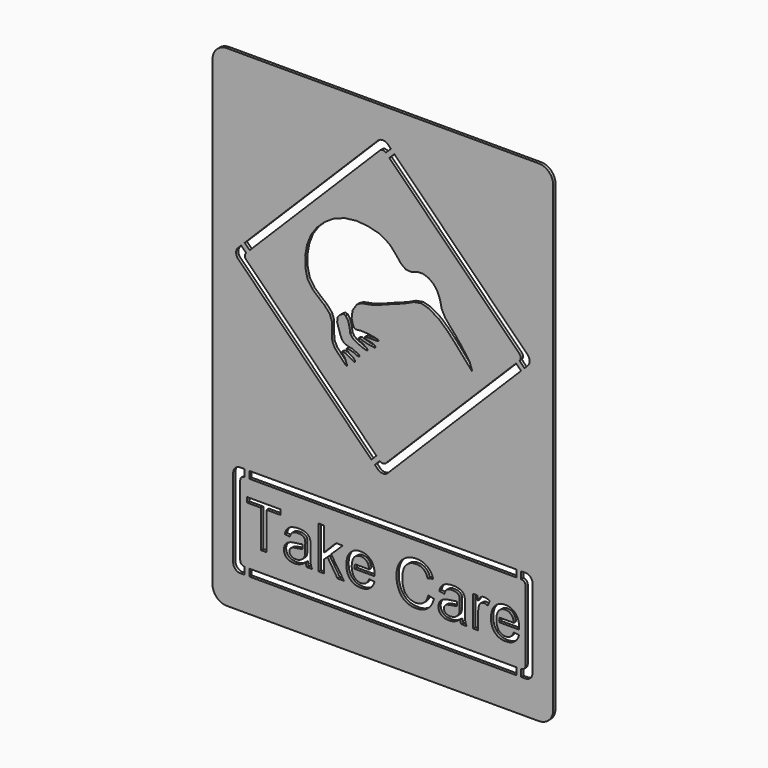
from build123d import *

# Parameters (mm, degrees)
F0_W     = 277.297216
F0_H     = 7.329178
F0_H_2   = 7.329177
F1_DEPTH = 3


# Not quite as in the source:
# - ends of sketch curves that miss each other by under 0.0002 mm in the source are joined


with BuildPart() as f1:
    # F0 (on Front) → F1 (new body)
    with BuildSketch(Plane.XZ):
        with BuildLine():
            Line((162.000001, 255), (-162, 255))
            ThreePointArc((-162, 255), (-172.6066017178, 250.6066027178), (-177, 240.000001))
            Line((-177, 240.000001), (-177, -240))
            ThreePointArc((-177, -240), (-172.6066017178, -250.6066017178), (-162, -255))
            Line((-162, -255), (162.000001, -255))
            ThreePointArc((162.000001, -255), (172.6066027178, -250.6066017178), (177.000001, -240))
            Line((177.000001, -240), (177, 240.000001))
            ThreePointArc((177, 240.000001), (172.6066027178, 250.6066027178), (162.000001, 255))
        make_face()
        with BuildLine():
            ThreePointArc((-148.146114, -208.902383), (-146.8581143129, -212.0118893129), (-143.748608, -213.299889))
            Line((-143.748608, -213.299889), (-143.748608, -220.629066))
            Line((-143.748608, -220.629066), (-148.146114, -220.629065))
            ThreePointArc((-148.146114, -220.629065), (-153.3286240501, -218.4823980501), (-155.47529, -213.299888))
            Line((-155.47529, -213.299888), (-155.47529, -131.21311))
            ThreePointArc((-155.47529, -131.21311), (-153.3286240501, -126.0305999499), (-148.146114, -123.883934))
            Line((-148.146114, -123.883934), (-143.748608, -123.883933))
            Line((-143.748608, -123.883933), (-143.748608, -131.21311))
            ThreePointArc((-143.748608, -131.21311), (-146.8581143129, -132.5011096871), (-148.146114, -135.610616))
            Line((-148.146114, -135.610616), (-148.146114, -208.902383))
        make_face(mode=Mode.SUBTRACT)
        Polygon((-120.79643, -153.786395), (-120.79643, -192.572038), (-126.615776, -192.572038), (-126.615776, -153.786395), (-141.104149, -153.786395), (-141.104149, -148.596979), (-106.248064, -148.596979), (-106.248064, -153.786395), align=None, mode=Mode.SUBTRACT)
        with Locations((0, -216.964477)):
            Rectangle(F0_W, F0_H, mode=Mode.SUBTRACT)
        Polygon((-80.02351, -189.731733), (-80.111626, -189.196011), (-80.180993, -188.64248), (-80.927393, -189.256473), (-81.666763, -189.823597), (-82.399102, -190.343851), (-83.124412, -190.817235), (-83.842691, -191.24375), (-84.553939, -191.623395), (-85.258156, -191.95617), (-85.955344, -192.242075), (-86.655343, -192.488142), (-87.367998, -192.701398), (-88.093306, -192.881848), (-88.831271, -193.029487), (-89.581889, -193.144318), (-90.345163, -193.22634), (-91.121092, -193.275553), (-91.909675, -193.291958), (-92.55636, -193.28194), (-93.184063, -193.251884), (-93.792784, -193.201792), (-94.382522, -193.131663), (-94.953279, -193.041497), (-95.505053, -192.931295), (-96.037844, -192.801056), (-96.551653, -192.65078), (-97.046481, -192.480466), (-97.522326, -192.290117), (-97.979188, -192.079731), (-98.417069, -191.849307), (-98.835967, -191.598847), (-99.235883, -191.32835), (-99.616817, -191.037816), (-99.978769, -190.727246), (-100.320215, -190.401091), (-100.639632, -190.063805), (-100.93702, -189.715386), (-101.21238, -189.355837), (-101.465711, -188.985156), (-101.697013, -188.603343), (-101.906286, -188.2104), (-102.093531, -187.806324), (-102.258747, -187.391116), (-102.401934, -186.964778), (-102.523092, -186.527307), (-102.622222, -186.078706), (-102.699323, -185.618972), (-102.754395, -185.148107), (-102.787438, -184.66611), (-102.798452, -184.172982), (-102.781813, -183.594375), (-102.731897, -183.028423), (-102.648703, -182.475126), (-102.532232, -181.934483), (-102.382483, -181.406496), (-102.199457, -180.891163), (-101.983152, -180.388485), (-101.733572, -179.898462), (-101.45704, -179.426719), (-101.159886, -178.978878), (-100.842109, -178.554941), (-100.50371, -178.154908), (-100.144687, -177.778778), (-99.765043, -177.426553), (-99.364775, -177.09823), (-98.943885, -176.793811), (-98.505888, -176.510249), (-98.054297, -176.244497), (-97.589115, -175.996557), (-97.110341, -175.766426), (-96.617975, -175.554106), (-96.112016, -175.359597), (-95.592465, -175.182898), (-95.059321, -175.02401), (-94.636556, -174.919491), (-94.163172, -174.815909), (-93.639168, -174.713263), (-93.064546, -174.611556), (-92.439303, -174.510786), (-91.763442, -174.410953), (-91.03696, -174.312058), (-90.259861, -174.2141), (-89.455927, -174.11544), (-88.678944, -174.014435), (-87.928911, -173.911088), (-87.205829, -173.805397), (-86.509696, -173.697362), (-85.840513, -173.586984), (-85.19828, -173.474262), (-84.582998, -173.359197), (-83.994666, -173.241788), (-83.685093, -173.175751), (-83.689838, -177.545451), (-83.765824, -177.564818), (-84.305529, -177.69371), (-84.8682, -177.819789), (-85.453838, -177.943057), (-86.062442, -178.063512), (-86.694011, -178.181155), (-87.348547, -178.295986), (-88.026049, -178.408005), (-88.726517, -178.517211), (-89.449951, -178.623605), (-90.251893, -178.745467), (-90.992903, -178.871078), (-91.672983, -179.000438), (-92.292132, -179.133548), (-92.850351, -179.270408), (-93.347639, -179.411017), (-93.783996, -179.555375), (-94.159422, -179.703484), (-94.494541, -179.862138), (-94.809974, -180.038134), (-95.105723, -180.231472), (-95.381785, -180.442151), (-95.638163, -180.670172), (-95.874855, -180.915535), (-96.091862, -181.17824), (-96.289183, -181.458287), (-96.464944, -181.750989), (-96.617271, -182.051658), (-96.746163, -182.360295), (-96.85162, -182.6769), (-96.933642, -183.001473), (-96.992229, -183.334013), (-97.027381, -183.674522), (-97.039099, -184.022999), (-97.013555, -184.551689), (-96.936923, -185.057883), (-96.809202, -185.541578), (-96.630394, -186.002776), (-96.400499, -186.441477), (-96.119515, -186.857681), (-95.787443, -187.251386), (-95.404283, -187.622594), (-94.971909, -187.960057), (-94.492198, -188.252524), (-93.965148, -188.499996), (-93.390759, -188.702473), (-92.769031, -188.859955), (-92.099966, -188.972443), (-91.383562, -189.039935), (-90.61982, -189.062433), (-89.850688, -189.041107), (-89.103116, -188.97713), (-88.377103, -188.870501), (-87.672651, -188.721221), (-86.989759, -188.529289), (-86.328427, -188.294707), (-85.688655, -188.017472), (-85.070444, -187.697586), (-84.483165, -187.340673), (-83.936195, -186.952357), (-83.429534, -186.532638), (-82.96318, -186.081518), (-82.537134, -185.598994), (-82.151396, -185.085067), (-81.805966, -184.539738), (-81.500844, -183.963005), (-81.296961, -183.478373), (-81.120262, -182.93937), (-80.970747, -182.345999), (-80.848418, -181.69826), (-80.753272, -180.996152), (-80.685311, -180.239674), (-80.644534, -179.428827), (-80.630943, -178.563612), (-80.623912, -172.089495), (-80.617818, -171.849991), (-80.612663, -171.635796), (-80.608444, -171.446912), (-80.605164, -171.283336), (-80.60282, -171.14507), (-80.601415, -171.032115), (-80.600945, -170.944468), (-80.606922, -170.539631), (-80.624849, -170.150026), (-80.654729, -169.775654), (-80.69656, -169.416515), (-80.750343, -169.072608), (-80.816078, -168.743934), (-80.893764, -168.430492), (-80.983402, -168.132284), (-81.084992, -167.849308), (-81.198535, -167.581565), (-81.324028, -167.329053), (-81.461473, -167.091776), (-81.610871, -166.86973), (-81.772221, -166.662918), (-81.945521, -166.471337), (-82.130774, -166.294991), (-82.397345, -166.073414), (-82.679619, -165.866132), (-82.977592, -165.673146), (-83.291268, -165.494455), (-83.620645, -165.330059), (-83.965723, -165.179959), (-84.326503, -165.044155), (-84.702984, -164.922644), (-85.095167, -164.81543), (-85.503051, -164.722511), (-85.926637, -164.643887), (-86.365923, -164.579558), (-86.82091, -164.529525), (-87.2916, -164.493786), (-87.777991, -164.472344), (-88.280083, -164.465195), (-88.748487, -164.47041), (-89.201308, -164.486053), (-89.638543, -164.512125), (-90.060195, -164.548624), (-90.466263, -164.595552), (-90.856746, -164.652909), (-91.231645, -164.720694), (-91.590961, -164.798909), (-91.934692, -164.887551), (-92.262839, -164.986621), (-92.575401, -165.096121), (-92.87238, -165.216049), (-93.153773, -165.346405), (-93.419583, -165.48719), (-93.66981, -165.638403), (-93.904451, -165.800046), (-94.127609, -165.974929), (-94.343386, -166.165864), (-94.55178, -166.372852), (-94.752794, -166.595894), (-94.946424, -166.834988), (-95.132672, -167.090136), (-95.311539, -167.361335), (-95.483024, -167.648588), (-95.647127, -167.951894), (-95.803847, -168.271253), (-95.953186, -168.606665), (-96.095142, -168.958129), (-96.229717, -169.325646), (-96.35691, -169.709216), (-96.476721, -170.108839), (-96.58915, -170.524516), (-101.868556, -169.804597), (-101.674046, -168.97758), (-101.450479, -168.19134), (-101.19785, -167.445877), (-100.916163, -166.74119), (-100.605417, -166.07728), (-100.265611, -165.454148), (-99.896746, -164.871791), (-99.498823, -164.330211), (-99.063402, -163.824018), (-98.58205, -163.347821), (-98.054766, -162.901621), (-97.48155, -162.485418), (-96.8624, -162.099212), (-96.197319, -161.743002), (-95.486304, -161.416789), (-94.729358, -161.120572), (-93.933979, -160.856929), (-93.107665, -160.628439), (-92.250418, -160.435102), (-91.362236, -160.276916), (-90.443121, -160.153883), (-89.493072, -160.066003), (-88.512088, -160.013274), (-87.50017, -159.995698), (-86.504188, -160.010696), (-85.556014, -160.055692), (-84.655646, -160.130683), (-83.803085, -160.235671), (-82.998332, -160.370656), (-82.241386, -160.535637), (-81.532247, -160.730615), (-80.870915, -160.95559), (-80.254578, -161.203297), (-79.680424, -161.46647), (-79.148452, -161.74511), (-78.658663, -162.039218), (-78.211058, -162.348793), (-77.805634, -162.673835), (-77.442394, -163.014343), (-77.121337, -163.370319), (-76.832619, -163.74598), (-76.566399, -164.145545), (-76.322676, -164.569012), (-76.101451, -165.016384), (-75.902723, -165.487659), (-75.726493, -165.982838), (-75.57276, -166.50192), (-75.441525, -167.044906), (-75.378251, -167.424551), (-75.323413, -167.873563), (-75.277012, -168.391942), (-75.239048, -168.979689), (-75.20952, -169.636802), (-75.188429, -170.363283), (-75.175773, -171.159131), (-75.171556, -172.024347), (-75.171556, -179.223538), (-75.170208, -180.143064), (-75.166165, -181.019352), (-75.159428, -181.852403), (-75.149995, -182.642217), (-75.137868, -183.388792), (-75.123046, -184.092131), (-75.105528, -184.752233), (-75.085315, -185.369098), (-75.062408, -185.942724), (-75.036805, -186.473114), (-75.008508, -186.960266), (-74.977515, -187.404181), (-74.943827, -187.804859), (-74.907444, -188.1623), (-74.868367, -188.476502), (-74.826594, -188.747468), (-74.729808, -189.243584), (-74.611931, -189.734545), (-74.472962, -190.220349), (-74.312901, -190.700999), (-74.13175, -191.176492), (-73.929508, -191.64683), (-73.706173, -192.112012), (-73.461747, -192.572038), (-79.101114, -192.572038), (-79.301716, -192.14318), (-79.483571, -191.696512), (-79.646677, -191.232032), (-79.791037, -190.749743), (-79.916648, -190.249643), align=None, mode=Mode.SUBTRACT)
        Polygon((-61.373106, -179.943457), (-61.373106, -192.572038), (-66.772499, -192.572038), (-66.772499, -148.596979), (-61.373106, -148.596979), (-61.373106, -173.674161), (-48.594541, -160.715617), (-41.605326, -160.715617), (-53.783958, -172.534289), (-40.375464, -192.572038), (-47.034716, -192.572038), (-57.563533, -176.283868), align=None, mode=Mode.SUBTRACT)
        with BuildLine():
            ThreePointArc((-29.2375033056, -178.0236729382), (-29.2848390712, -175.7969741165), (-29.0319847673, -173.5841720427))
            Line((-29.0319847673, -173.5841720427), (-14.218403, -173.584172))
            Line((-14.218403, -173.584172), (-14.268553, -173.089579))
            Line((-14.268553, -173.089579), (-14.329015, -172.610687))
            Line((-14.329015, -172.610687), (-14.399788, -172.147497))
            Line((-14.399788, -172.147497), (-14.480873, -171.700008))
            Line((-14.480873, -171.700008), (-14.572269, -171.268221))
            Line((-14.572269, -171.268221), (-14.673977, -170.852134))
            Line((-14.673977, -170.852134), (-14.785995, -170.45175))
            Line((-14.785995, -170.45175), (-14.908325, -170.067067))
            Line((-14.908325, -170.067067), (-15.040966, -169.698084))
            Line((-15.040966, -169.698084), (-15.183919, -169.344804))
            Line((-15.183919, -169.344804), (-15.337183, -169.007225))
            Line((-15.337183, -169.007225), (-15.500758, -168.685346))
            Line((-15.500758, -168.685346), (-15.674646, -168.37917))
            Line((-15.674646, -168.37917), (-15.858843, -168.088695))
            Line((-15.858843, -168.088695), (-16.053352, -167.813922))
            Line((-16.053352, -167.813922), (-16.258173, -167.554849))
            Line((-16.258173, -167.554849), (-16.586613, -167.177079))
            Line((-16.586613, -167.177079), (-16.927005, -166.823681))
            Line((-16.927005, -166.823681), (-17.279347, -166.494656))
            Line((-17.279347, -166.494656), (-17.643642, -166.190002))
            Line((-17.643642, -166.190002), (-18.01989, -165.909721))
            Line((-18.01989, -165.909721), (-18.408088, -165.653813))
            Line((-18.408088, -165.653813), (-18.808239, -165.422276))
            Line((-18.808239, -165.422276), (-19.220341, -165.215112))
            Line((-19.220341, -165.215112), (-19.644395, -165.032319))
            Line((-19.644395, -165.032319), (-20.0804, -164.8739))
            Line((-20.0804, -164.8739), (-20.528357, -164.739853))
            Line((-20.528357, -164.739853), (-20.988267, -164.630177))
            Line((-20.988267, -164.630177), (-21.460128, -164.544875))
            Line((-21.460128, -164.544875), (-21.943941, -164.483944))
            Line((-21.943941, -164.483944), (-22.439706, -164.447385))
            Line((-22.439706, -164.447385), (-22.947422, -164.435199))
            Line((-22.947422, -164.435199), (-23.407741, -164.444925))
            Line((-23.407741, -164.444925), (-23.858804, -164.474101))
            Line((-23.858804, -164.474101), (-24.30061, -164.522728))
            Line((-24.30061, -164.522728), (-24.733158, -164.590806))
            Line((-24.733158, -164.590806), (-25.156451, -164.678336))
            Line((-25.156451, -164.678336), (-25.570487, -164.785316))
            Line((-25.570487, -164.785316), (-25.975265, -164.911747))
            Line((-25.975265, -164.911747), (-26.370788, -165.05763))
            Line((-26.370788, -165.05763), (-26.757053, -165.222963))
            Line((-26.757053, -165.222963), (-27.134061, -165.407746))
            Line((-27.134061, -165.407746), (-27.501813, -165.611981))
            Line((-27.501813, -165.611981), (-27.860307, -165.835667))
            Line((-27.860307, -165.835667), (-28.209546, -166.078804))
            Line((-28.209546, -166.078804), (-28.549527, -166.341392))
            Line((-28.549527, -166.341392), (-28.880252, -166.62343))
            Line((-28.880252, -166.62343), (-29.201719, -166.924919))
            Line((-29.201719, -166.924919), (-29.509712, -167.242696))
            Line((-29.509712, -167.242696), (-29.800011, -167.573596))
            Line((-29.800011, -167.573596), (-30.072618, -167.917621))
            Line((-30.072618, -167.917621), (-30.32753, -168.274768))
            Line((-30.32753, -168.274768), (-30.564749, -168.645039))
            Line((-30.564749, -168.645039), (-30.784276, -169.028434))
            Line((-30.784276, -169.028434), (-30.986108, -169.424952))
            Line((-30.986108, -169.424952), (-31.170248, -169.834593))
            ThreePointArc((-31.170248, -169.834593), (-32.3623662835, -176.4885053369), (-31.2191093274, -183.1509867594))
            Line((-31.2191093274, -183.1509867594), (-30.773847, -184.079008))
            Line((-30.773847, -184.079008), (-30.523445, -184.514194))
            Line((-30.523445, -184.514194), (-30.254531, -184.930162))
            Line((-30.254531, -184.930162), (-29.967102, -185.326915))
            Line((-29.967102, -185.326915), (-29.66116, -185.70445))
            Line((-29.66116, -185.70445), (-29.336704, -186.062769))
            Line((-29.336704, -186.062769), (-28.997836, -186.400583))
            Line((-28.997836, -186.400583), (-28.648657, -186.716603))
            Line((-28.648657, -186.716603), (-28.289166, -187.010828))
            Line((-28.289166, -187.010828), (-27.919363, -187.283257))
            Line((-27.919363, -187.283257), (-27.53925, -187.533894))
            Line((-27.53925, -187.533894), (-27.148824, -187.762735))
            Line((-27.148824, -187.762735), (-26.748089, -187.969782))
            Line((-26.748089, -187.969782), (-26.337041, -188.155035))
            Line((-26.337041, -188.155035), (-25.915682, -188.318493))
            Line((-25.915682, -188.318493), (-25.484012, -188.460157))
            Line((-25.484012, -188.460157), (-25.042031, -188.580026))
            Line((-25.042031, -188.580026), (-24.589737, -188.678101))
            Line((-24.589737, -188.678101), (-24.127134, -188.754381))
            Line((-24.127134, -188.754381), (-23.654218, -188.808867))
            Line((-23.654218, -188.808867), (-23.170991, -188.841559))
            Line((-23.170991, -188.841559), (-22.677452, -188.852456))
            Line((-22.677452, -188.852456), (-21.948628, -188.828084))
            Line((-21.948628, -188.828084), (-21.246988, -188.754967))
            Line((-21.246988, -188.754967), (-20.572533, -188.633106))
            Line((-20.572533, -188.633106), (-19.925261, -188.4625))
            Line((-19.925261, -188.4625), (-19.305174, -188.24315))
            Line((-19.305174, -188.24315), (-18.712273, -187.975055))
            Line((-18.712273, -187.975055), (-18.146555, -187.658216))
            Line((-18.146555, -187.658216), (-17.608022, -187.292631))
            Line((-17.608022, -187.292631), (-17.096672, -186.873616))
            Line((-17.096672, -186.873616), (-16.612509, -186.396483))
            Line((-16.612509, -186.396483), (-16.155529, -185.861229))
            Line((-16.155529, -185.861229), (-15.725733, -185.267859))
            Line((-15.725733, -185.267859), (-15.323122, -184.616369))
            Line((-15.323122, -184.616369), (-14.947696, -183.906762))
            Line((-14.947696, -183.906762), (-14.599453, -183.139035))
            Line((-14.599453, -183.139035), (-14.278396, -182.313191))
            Line((-14.278396, -182.313191), (-8.699023, -183.003113))
            Line((-8.699023, -183.003113), (-8.872792, -183.605741))
            Line((-8.872792, -183.605741), (-9.064138, -184.191261))
            Line((-9.064138, -184.191261), (-9.273059, -184.759674))
            Line((-9.273059, -184.759674), (-9.499557, -185.310979))
            Line((-9.499557, -185.310979), (-9.743632, -185.845177))
            Line((-9.743632, -185.845177), (-10.005281, -186.362268))
            Line((-10.005281, -186.362268), (-10.284509, -186.86225))
            Line((-10.284509, -186.86225), (-10.581311, -187.345125))
            Line((-10.581311, -187.345125), (-10.895689, -187.810893))
            Line((-10.895689, -187.810893), (-11.227644, -188.259554))
            Line((-11.227644, -188.259554), (-11.577176, -188.691107))
            Line((-11.577176, -188.691107), (-11.944283, -189.105553))
            Line((-11.944283, -189.105553), (-12.328966, -189.502891))
            Line((-12.328966, -189.502891), (-12.731225, -189.883122))
            Line((-12.731225, -189.883122), (-13.151061, -190.246245))
            Line((-13.151061, -190.246245), (-13.588473, -190.592261))
            Line((-13.588473, -190.592261), (-14.042407, -190.919177))
            Line((-14.042407, -190.919177), (-14.511807, -191.225003))
            Line((-14.511807, -191.225003), (-14.996674, -191.509736))
            Line((-14.996674, -191.509736), (-15.497008, -191.773378))
            Line((-15.497008, -191.773378), (-16.01281, -192.015929))
            Line((-16.01281, -192.015929), (-16.544078, -192.237388))
            Line((-16.544078, -192.237388), (-17.090815, -192.437757))
            Line((-17.090815, -192.437757), (-17.653017, -192.617033))
            Line((-17.653017, -192.617033), (-18.230686, -192.775219))
            Line((-18.230686, -192.775219), (-18.823823, -192.912313))
            Line((-18.823823, -192.912313), (-19.432426, -193.028316))
            Line((-19.432426, -193.028316), (-20.056496, -193.123227))
            Line((-20.056496, -193.123227), (-20.696034, -193.197046))
            Line((-20.696034, -193.197046), (-21.351038, -193.249775))
            Line((-21.351038, -193.249775), (-22.02151, -193.281412))
            Line((-22.02151, -193.281412), (-22.707449, -193.291958))
            Line((-22.707449, -193.291958), (-23.569793, -193.275143))
            Line((-23.569793, -193.275143), (-24.409524, -193.224699))
            Line((-24.409524, -193.224699), (-25.226638, -193.140627))
            Line((-25.226638, -193.140627), (-26.021139, -193.022925))
            Line((-26.021139, -193.022925), (-26.793025, -192.871595))
            Line((-26.793025, -192.871595), (-27.542297, -192.686635))
            Line((-27.542297, -192.686635), (-28.268953, -192.468046))
            Line((-28.268953, -192.468046), (-28.972995, -192.215828))
            Line((-28.972995, -192.215828), (-29.654423, -191.929982))
            Line((-29.654423, -191.929982), (-30.313235, -191.610505))
            Line((-30.313235, -191.610505), (-30.949433, -191.257401))
            Line((-30.949433, -191.257401), (-31.563016, -190.870667))
            Line((-31.563016, -190.870667), (-32.153985, -190.450304))
            Line((-32.153985, -190.450304), (-32.722339, -189.996313))
            Line((-32.722339, -189.996313), (-33.268079, -189.508691))
            Line((-33.268079, -189.508691), (-33.791204, -188.987441))
            Line((-33.791204, -188.987441), (-34.287027, -188.435843))
            Line((-34.287027, -188.435843), (-34.750862, -187.857178))
            Line((-34.750862, -187.857178), (-35.182708, -187.251445))
            Line((-35.182708, -187.251445), (-35.582565, -186.618645))
            Line((-35.582565, -186.618645), (-35.950434, -185.958777))
            Line((-35.950434, -185.958777), (-36.286314, -185.271843))
            Line((-36.286314, -185.271843), (-36.590206, -184.557841))
            Line((-36.590206, -184.557841), (-36.862109, -183.816772))
            Line((-36.862109, -183.816772), (-37.102023, -183.048636))
            Line((-37.102023, -183.048636), (-37.309949, -182.253432))
            Line((-37.309949, -182.253432), (-37.485886, -181.431161))
            Line((-37.485886, -181.431161), (-37.629835, -180.581823))
            Line((-37.629835, -180.581823), (-37.741795, -179.705417))
            Line((-37.741795, -179.705417), (-37.821767, -178.801945))
            Line((-37.821767, -178.801945), (-37.86975, -177.871404))
            Line((-37.86975, -177.871404), (-37.885744, -176.913798))
            Line((-37.885744, -176.913798), (-37.869574, -175.922972))
            Line((-37.869574, -175.922972), (-37.821064, -174.960267))
            Line((-37.821064, -174.960267), (-37.740214, -174.025684))
            Line((-37.740214, -174.025684), (-37.627023, -173.119223))
            Line((-37.627023, -173.119223), (-37.481493, -172.240885))
            Line((-37.481493, -172.240885), (-37.303622, -171.390668))
            Line((-37.303622, -171.390668), (-37.093411, -170.568572))
            Line((-37.093411, -170.568572), (-36.85086, -169.774599))
            Line((-36.85086, -169.774599), (-36.575969, -169.008748))
            Line((-36.575969, -169.008748), (-36.268738, -168.271018))
            Line((-36.268738, -168.271018), (-35.929167, -167.56141))
            Line((-35.929167, -167.56141), (-35.557256, -166.879925))
            Line((-35.557256, -166.879925), (-35.153004, -166.226561))
            Line((-35.153004, -166.226561), (-34.716413, -165.601318))
            Line((-34.716413, -165.601318), (-34.247481, -165.004198))
            Line((-34.247481, -165.004198), (-33.746209, -164.435199))
            Line((-33.746209, -164.435199), (-33.219159, -163.897603))
            Line((-33.219159, -163.897603), (-32.672891, -163.394691))
            Line((-32.672891, -163.394691), (-32.107409, -162.926462))
            Line((-32.107409, -162.926462), (-31.522709, -162.492917))
            Line((-31.522709, -162.492917), (-30.918792, -162.094055))
            Line((-30.918792, -162.094055), (-30.295659, -161.729878))
            Line((-30.295659, -161.729878), (-29.653309, -161.400384))
            Line((-29.653309, -161.400384), (-28.991743, -161.105573))
            Line((-28.991743, -161.105573), (-28.31096, -160.845446))
            Line((-28.31096, -160.845446), (-27.610961, -160.620002))
            Line((-27.610961, -160.620002), (-26.891745, -160.429243))
            Line((-26.891745, -160.429243), (-26.153312, -160.273167))
            Line((-26.153312, -160.273167), (-25.395663, -160.151774))
            Line((-25.395663, -160.151774), (-24.618797, -160.065065))
            Line((-24.618797, -160.065065), (-23.822715, -160.01304))
            Line((-23.822715, -160.01304), (-23.007415, -159.995698))
            Line((-23.007415, -159.995698), (-22.217895, -160.012688))
            Line((-22.217895, -160.012688), (-21.446653, -160.063659))
            Line((-21.446653, -160.063659), (-20.693691, -160.14861))
            Line((-20.693691, -160.14861), (-19.959008, -160.267542))
            Line((-19.959008, -160.267542), (-19.242603, -160.420455))
            Line((-19.242603, -160.420455), (-18.544479, -160.607348))
            Line((-18.544479, -160.607348), (-17.864633, -160.828221))
            Line((-17.864633, -160.828221), (-17.203068, -161.083075))
            Line((-17.203068, -161.083075), (-16.55978, -161.371911))
            Line((-16.55978, -161.371911), (-15.934772, -161.694725))
            Line((-15.934772, -161.694725), (-15.328043, -162.051521))
            Line((-15.328043, -162.051521), (-14.739594, -162.442298))
            Line((-14.739594, -162.442298), (-14.169423, -162.867055))
            Line((-14.169423, -162.867055), (-13.617533, -163.325792))
            Line((-13.617533, -163.325792), (-13.083921, -163.81851))
            Line((-13.083921, -163.81851), (-12.568587, -164.34521))
            Line((-12.568587, -164.34521), (-12.078213, -164.902724))
            Line((-12.078213, -164.902724), (-11.619475, -165.487893))
            Line((-11.619475, -165.487893), (-11.192375, -166.100715))
            Line((-11.192375, -166.100715), (-10.796912, -166.74119))
            Line((-10.796912, -166.74119), (-10.433086, -167.409318))
            Line((-10.433086, -167.409318), (-10.100896, -168.105099))
            Line((-10.100896, -168.105099), (-9.800344, -168.828534))
            Line((-9.800344, -168.828534), (-9.531429, -169.579621))
            Line((-9.531429, -169.579621), (-9.294151, -170.358362))
            Line((-9.294151, -170.358362), (-9.08851, -171.164755))
            Line((-9.08851, -171.164755), (-8.914506, -171.998802))
            Line((-8.914506, -171.998802), (-8.772139, -172.860502))
            Line((-8.772139, -172.860502), (-8.661409, -173.749856))
            Line((-8.661409, -173.749856), (-8.582317, -174.666862))
            Line((-8.582317, -174.666862), (-8.534862, -175.611522))
            Line((-8.534862, -175.611522), (-8.519043, -176.583835))
            Line((-8.519043, -176.583835), (-8.520917, -176.853804))
            Line((-8.520917, -176.853804), (-8.526542, -177.183767))
            Line((-8.526542, -177.183767), (-8.535915, -177.573723))
            Line((-8.535915, -177.573723), (-8.54904, -178.023673))
            Line((-8.54904, -178.023673), (-29.2375033056, -178.0236729382))
        make_face(mode=Mode.SUBTRACT)
        with Locations((0, -127.5485215)):
            Rectangle(F0_W, F0_H_2, mode=Mode.SUBTRACT)
        Polygon((46.880515, -178.498464), (47.056159, -177.836779), (47.214697, -177.15377), (53.034043, -178.623605), (52.793894, -179.506455), (52.530896, -180.362707), (52.245049, -181.19236), (51.936353, -181.995414), (51.604809, -182.77187), (51.250415, -183.521727), (50.873172, -184.244985), (50.473081, -184.941645), (50.05014, -185.611707), (49.60435, -186.25517), (49.135711, -186.872034), (48.644223, -187.4623), (48.129887, -188.025967), (47.592701, -188.563036), (47.032666, -189.073505), (46.449783, -189.557377), (45.847214, -190.013244), (45.228123, -190.439699), (44.592511, -190.836745), (43.940377, -191.204379), (43.271722, -191.542603), (42.586545, -191.851416), (41.884846, -192.130819), (41.166626, -192.38081), (40.431885, -192.601391), (39.680621, -192.792561), (38.912836, -192.95432), (38.12853, -193.086668), (37.327701, -193.189606), (36.510352, -193.263133), (35.67648, -193.307249), (34.826088, -193.321954), (33.947808, -193.310647), (33.090267, -193.276725), (32.253466, -193.220188), (31.437406, -193.141037), (30.642086, -193.039271), (29.867505, -192.914891), (29.113664, -192.767895), (28.380562, -192.598286), (27.668201, -192.406061), (26.976579, -192.191222), (26.305698, -191.953768), (25.655556, -191.6937), (25.026153, -191.411017), (24.417492, -191.105719), (23.82957, -190.777806), (23.262387, -190.427279), (22.713894, -190.055309), (22.18204, -189.663068), (21.666824, -189.250556), (21.168247, -188.817773), (20.686309, -188.364719), (20.22101, -187.891393), (19.77235, -187.397795), (19.340328, -186.883927), (18.924945, -186.349788), (18.5262, -185.795378), (18.144095, -185.220696), (17.778628, -184.625743), (17.4298, -184.01052), (17.097611, -183.375024), (16.782061, -182.719258), (16.483149, -182.043222), (16.201638, -181.353884), (15.938288, -180.658221), (15.6931, -179.956229), (15.466076, -179.247911), (15.257213, -178.533264), (15.066511, -177.81229), (14.893972, -177.084989), (14.739594, -176.35136), (14.603379, -175.611405), (14.485327, -174.865122), (14.385435, -174.11251), (14.303706, -173.353572), (14.240139, -172.588307), (14.194734, -171.816714), (14.16749, -171.038793), (14.158409, -170.254545), (14.168662, -169.402747), (14.199421, -168.564657), (14.250685, -167.740277), (14.322454, -166.929606), (14.414728, -166.132645), (14.527509, -165.349394), (14.660795, -164.579851), (14.814587, -163.824018), (14.988883, -163.081894), (15.183685, -162.35348), (15.398994, -161.638775), (15.634806, -160.937779), (15.891125, -160.250493), (16.16795, -159.576917), (16.465279, -158.917049), (16.783115, -158.270891), (17.119874, -157.641196), (17.473975, -157.030718), (17.845418, -156.439457), (18.234202, -155.867411), (18.640328, -155.314584), (19.063796, -154.780972), (19.504606, -154.266575), (19.962758, -153.771397), (20.438252, -153.295435), (20.931087, -152.83869), (21.441263, -152.401161), (21.968782, -151.982848), (22.513644, -151.583752), (23.075845, -151.203873), (23.65539, -150.843211), (24.252276, -150.501765), (24.861641, -150.180296), (25.478622, -149.879569), (26.10322, -149.599581), (26.735435, -149.340332), (27.375265, -149.101824), (28.022712, -148.884056), (28.677775, -148.687026), (29.340455, -148.510738), (30.010751, -148.355189), (30.688662, -148.22038), (31.374191, -148.106311), (32.067336, -148.012982), (32.768096, -147.940392), (33.476474, -147.888542), (34.192468, -147.857433), (34.916078, -147.847063), (35.732783, -147.860186), (36.533084, -147.899557), (37.31698, -147.965175), (38.084472, -148.057039), (38.835559, -148.175151), (39.570243, -148.319509), (40.288522, -148.490115), (40.990396, -148.686968), (41.675865, -148.910068), (42.344931, -149.159415), (42.997592, -149.435009), (43.633848, -149.73685), (44.253701, -150.064938), (44.857149, -150.419274), (45.444192, -150.799856), (46.014831, -151.206686), (46.566605, -151.637301), (47.097053, -152.089243), (47.606176, -152.562509), (48.093973, -153.057102), (48.560444, -153.573021), (49.00559, -154.110266), (49.429409, -154.668835), (49.831903, -155.248731), (50.213071, -155.849953), (50.572913, -156.4725), (50.91143, -157.116373), (51.22862, -157.781572), (51.524486, -158.468096), (51.799025, -159.175947), (52.052239, -159.905122), (52.284127, -160.655624), (46.55477, -162.005473), (46.358152, -161.415734), (46.150753, -160.846383), (45.932575, -160.297422), (45.703616, -159.768848), (45.463877, -159.260664), (45.213359, -158.772866), (44.95206, -158.305458), (44.679982, -157.858438), (44.397122, -157.431806), (44.103484, -157.025563), (43.799065, -156.639707), (43.483865, -156.274241), (43.157887, -155.929162), (42.821128, -155.604473), (42.473588, -155.300171), (42.115269, -155.016257), (41.745702, -154.751092), (41.364417, -154.503034), (40.971414, -154.272083), (40.566693, -154.058239), (40.150256, -153.861504), (39.7221, -153.681876), (39.282228, -153.519355), (38.830639, -153.373942), (38.367331, -153.245636), (37.892306, -153.134438), (37.405564, -153.040347), (36.907104, -152.963363), (36.396927, -152.903487), (35.875033, -152.860719), (35.341421, -152.835057), (34.796092, -152.826504), (34.168916, -152.835995), (33.554747, -152.864468), (32.953583, -152.911924), (32.365427, -152.978361), (31.790277, -153.063781), (31.228133, -153.168183), (30.678996, -153.291569), (30.142864, -153.433935), (29.61974, -153.595284), (29.10962, -153.775616), (28.612509, -153.974929), (28.128403, -154.193225), (27.657304, -154.430503), (27.19921, -154.686763), (26.754124, -154.962005), (26.322043, -155.25623), (25.904376, -155.566449), (25.502526, -155.889675), (25.116495, -156.225907), (24.746283, -156.575144), (24.391889, -156.937389), (24.053314, -157.31264), (23.730558, -157.700897), (23.423619, -158.102161), (23.132499, -158.516431), (22.857198, -158.943707), (22.597716, -159.383989), (22.354051, -159.837278), (22.126206, -160.303574), (21.914179, -160.782875), (21.717971, -161.275183), (21.537581, -161.780497), (21.21418, -162.808117), (20.933899, -163.843703), (20.696738, -164.887258), (20.502697, -165.93878), (20.351777, -166.998271), (20.243976, -168.065729), (20.179296, -169.141155), (20.157736, -170.224549), (20.18328, -171.604628), (20.259912, -172.940182), (20.387632, -174.231208), (20.56644, -175.477709), (20.796336, -176.679683), (21.07732, -177.837131), (21.409393, -178.950053), (21.792553, -180.018449), (22.003993, -180.533254), (22.229612, -181.031538), (22.46941, -181.5133), (22.723385, -181.978541), (22.991539, -182.42726), (23.27387, -182.859457), (23.57038, -183.275134), (23.881068, -183.674288), (24.205934, -184.056921), (24.544978, -184.423032), (24.8982, -184.772621), (25.265599, -185.10569), (25.647177, -185.422236), (26.042934, -185.722261), (26.452868, -186.005765), (26.876981, -186.272746), (27.74829, -186.757848), (28.637408, -187.17827), (29.544337, -187.534011), (30.469077, -187.825071), (31.411628, -188.051452), (32.371988, -188.213153), (33.35016, -188.310173), (34.346142, -188.342513), (34.951464, -188.331499), (35.54507, -188.298456), (36.126957, -188.243384), (36.697128, -188.166284), (37.255581, -188.067154), (37.802316, -187.945995), (38.337334, -187.802809), (38.860635, -187.637593), (39.372218, -187.450348), (39.872084, -187.241075), (40.360232, -187.009773), (40.836662, -186.756442), (41.301377, -186.481082), (41.754373, -186.183693), (42.195651, -185.864276), (42.625212, -185.52283), (43.04036, -185.159707), (43.438402, -184.775258), (43.819335, -184.369484), (44.183162, -183.942383), (44.529881, -183.493956), (44.859493, -183.024205), (45.171996, -182.533128), (45.467393, -182.020723), (45.745682, -181.486994), (46.006863, -180.93194), (46.250938, -180.355559), (46.477904, -179.757852), (46.687764, -179.138821), align=None, mode=Mode.SUBTRACT)
        Polygon((80.458463, -189.731733), (80.370347, -189.196011), (80.30098, -188.64248), (79.554579, -189.256473), (78.815209, -189.823597), (78.082869, -190.343851), (77.357561, -190.817235), (76.639282, -191.24375), (75.928034, -191.623395), (75.223815, -191.95617), (74.526628, -192.242075), (73.826629, -192.488142), (73.113975, -192.701398), (72.388665, -192.881848), (71.650701, -193.029487), (70.900082, -193.144318), (70.136809, -193.22634), (69.360881, -193.275553), (68.572298, -193.291958), (67.925612, -193.28194), (67.29791, -193.251884), (66.689189, -193.201792), (66.09945, -193.131663), (65.528694, -193.041497), (64.97692, -192.931295), (64.444128, -192.801056), (63.930318, -192.65078), (63.435492, -192.480466), (62.959647, -192.290117), (62.502783, -192.079731), (62.064904, -191.849307), (61.646005, -191.598847), (61.246089, -191.32835), (60.865155, -191.037816), (60.503204, -190.727246), (60.161758, -190.401091), (59.842341, -190.063805), (59.544952, -189.715386), (59.269593, -189.355837), (59.016261, -188.985156), (58.784959, -188.603343), (58.575685, -188.2104), (58.388441, -187.806324), (58.223226, -187.391116), (58.080039, -186.964778), (57.95888, -186.527307), (57.859751, -186.078706), (57.78265, -185.618972), (57.727578, -185.148107), (57.694535, -184.66611), (57.68352, -184.172982), (57.700159, -183.594375), (57.750075, -183.028423), (57.833269, -182.475126), (57.949741, -181.934483), (58.099489, -181.406496), (58.282516, -180.891163), (58.498819, -180.388485), (58.748401, -179.898462), (59.024932, -179.426719), (59.322087, -178.978878), (59.639864, -178.554941), (59.978263, -178.154908), (60.337285, -177.778778), (60.71693, -177.426553), (61.117197, -177.09823), (61.538088, -176.793811), (61.976085, -176.510249), (62.427675, -176.244497), (62.892857, -175.996557), (63.371632, -175.766426), (63.863998, -175.554106), (64.369957, -175.359597), (64.889508, -175.182898), (65.422651, -175.02401), (65.845416, -174.919491), (66.3188, -174.815909), (66.842804, -174.713263), (67.417427, -174.611556), (68.04267, -174.510786), (68.718531, -174.410953), (69.445012, -174.312058), (70.222112, -174.2141), (71.026045, -174.11544), (71.803028, -174.014435), (72.553061, -173.911088), (73.276144, -173.805397), (73.972276, -173.697362), (74.64146, -173.586984), (75.283691, -173.474262), (75.898974, -173.359197), (76.487307, -173.241788), (76.79688, -173.175751), (76.792134, -177.545451), (76.716148, -177.564818), (76.176443, -177.69371), (75.613772, -177.819789), (75.028135, -177.943057), (74.419531, -178.063512), (73.787961, -178.181155), (73.133425, -178.295986), (72.455923, -178.408005), (71.755455, -178.517211), (71.032021, -178.623605), (70.23008, -178.745467), (69.489069, -178.871078), (68.80899, -179.000438), (68.18984, -179.133548), (67.631622, -179.270408), (67.134334, -179.411017), (66.697976, -179.555375), (66.32255, -179.703484), (65.987432, -179.862138), (65.671998, -180.038134), (65.37625, -180.231472), (65.100187, -180.442151), (64.84381, -180.670172), (64.607118, -180.915535), (64.390111, -181.17824), (64.192789, -181.458287), (64.017027, -181.750989), (63.864701, -182.051658), (63.735809, -182.360295), (63.630353, -182.6769), (63.54833, -183.001473), (63.489744, -183.334013), (63.454591, -183.674522), (63.442874, -184.022999), (63.468417, -184.551689), (63.54505, -185.057883), (63.672769, -185.541578), (63.851577, -186.002776), (64.081474, -186.441477), (64.362458, -186.857681), (64.69453, -187.251386), (65.07769, -187.622594), (65.510063, -187.960057), (65.989775, -188.252524), (66.516825, -188.499996), (67.091214, -188.702473), (67.71294, -188.859955), (68.382006, -188.972443), (69.09841, -189.039935), (69.862153, -189.062433), (70.631285, -189.041107), (71.378857, -188.97713), (72.10487, -188.870501), (72.809321, -188.721221), (73.492213, -188.529289), (74.153546, -188.294707), (74.793317, -188.017472), (75.411529, -187.697586), (75.998806, -187.340673), (76.545776, -186.952357), (77.052439, -186.532638), (77.518792, -186.081518), (77.944838, -185.598994), (78.330576, -185.085067), (78.676006, -184.539738), (78.981128, -183.963005), (79.185011, -183.478373), (79.361711, -182.93937), (79.511224, -182.345999), (79.633555, -181.69826), (79.728701, -180.996152), (79.796661, -180.239674), (79.837438, -179.428827), (79.85103, -178.563612), (79.858061, -172.089495), (79.864153, -171.849991), (79.86931, -171.635796), (79.873528, -171.446912), (79.876809, -171.283336), (79.879153, -171.14507), (79.880558, -171.032115), (79.881027, -170.944468), (79.875051, -170.539631), (79.857124, -170.150026), (79.827244, -169.775654), (79.785413, -169.416515), (79.73163, -169.072608), (79.665895, -168.743934), (79.588209, -168.430492), (79.49857, -168.132284), (79.39698, -167.849308), (79.283438, -167.581565), (79.157944, -167.329053), (79.020498, -167.091776), (78.871101, -166.86973), (78.709752, -166.662918), (78.536451, -166.471337), (78.351199, -166.294991), (78.084627, -166.073414), (77.802354, -165.866132), (77.504379, -165.673146), (77.190704, -165.494455), (76.861328, -165.330059), (76.516248, -165.179959), (76.155469, -165.044155), (75.778988, -164.922644), (75.386805, -164.81543), (74.978922, -164.722511), (74.555336, -164.643887), (74.11605, -164.579558), (73.661061, -164.529525), (73.190372, -164.493786), (72.703982, -164.472344), (72.20189, -164.465195), (71.733486, -164.47041), (71.280665, -164.486053), (70.843428, -164.512125), (70.421777, -164.548624), (70.01571, -164.595552), (69.625226, -164.652909), (69.250326, -164.720694), (68.891012, -164.798909), (68.547281, -164.887551), (68.219134, -164.986621), (67.906571, -165.096121), (67.609593, -165.216049), (67.328198, -165.346405), (67.062388, -165.48719), (66.812163, -165.638403), (66.577521, -165.800046), (66.354363, -165.974929), (66.138587, -166.165864), (65.930192, -166.372852), (65.729179, -166.595894), (65.535548, -166.834988), (65.3493, -167.090136), (65.170433, -167.361335), (64.998949, -167.648588), (64.834846, -167.951894), (64.678125, -168.271253), (64.528787, -168.606665), (64.386829, -168.958129), (64.252255, -169.325646), (64.125063, -169.709216), (64.005252, -170.108839), (63.892823, -170.524516), (58.613416, -169.804597), (58.807925, -168.97758), (59.031494, -168.19134), (59.284122, -167.445877), (59.565809, -166.74119), (59.876556, -166.07728), (60.216361, -165.454148), (60.585226, -164.871791), (60.98315, -164.330211), (61.418569, -163.824018), (61.899922, -163.347821), (62.427207, -162.901621), (63.000423, -162.485418), (63.619572, -162.099212), (64.284654, -161.743002), (64.995668, -161.416789), (65.752614, -161.120572), (66.547993, -160.856929), (67.374306, -160.628439), (68.231554, -160.435102), (69.119736, -160.276916), (70.038851, -160.153883), (70.988901, -160.066003), (71.969885, -160.013274), (72.981802, -159.995698), (73.977783, -160.010696), (74.925958, -160.055692), (75.826326, -160.130683), (76.678886, -160.235671), (77.48364, -160.370656), (78.240586, -160.535637), (78.949726, -160.730615), (79.611057, -160.95559), (80.227394, -161.203297), (80.801549, -161.46647), (81.33352, -161.74511), (81.823308, -162.039218), (82.270915, -162.348793), (82.676338, -162.673835), (83.039579, -163.014343), (83.360636, -163.370319), (83.649354, -163.74598), (83.915574, -164.145545), (84.159296, -164.569012), (84.380522, -165.016384), (84.579249, -165.487659), (84.75548, -165.982838), (84.909212, -166.50192), (85.040447, -167.044906), (85.103721, -167.424551), (85.158559, -167.873563), (85.20496, -168.391942), (85.242925, -168.979689), (85.272453, -169.636802), (85.293544, -170.363283), (85.306199, -171.159131), (85.310417, -172.024347), (85.310417, -179.223538), (85.311764, -180.143064), (85.315807, -181.019352), (85.322545, -181.852403), (85.331977, -182.642217), (85.344105, -183.388792), (85.358927, -184.092131), (85.376445, -184.752233), (85.396657, -185.369098), (85.419565, -185.942724), (85.445167, -186.473114), (85.473465, -186.960266), (85.504458, -187.404181), (85.538145, -187.804859), (85.574528, -188.1623), (85.613606, -188.476502), (85.655378, -188.747468), (85.752165, -189.243584), (85.870042, -189.734545), (86.009011, -190.220349), (86.16907, -190.700999), (86.350222, -191.176492), (86.552465, -191.64683), (86.775799, -192.112012), (87.020225, -192.572038), (81.380859, -192.572038), (81.180256, -192.14318), (80.998402, -191.696512), (80.835294, -191.232032), (80.690936, -190.749743), (80.565325, -190.249643), align=None, mode=Mode.SUBTRACT)
        Polygon((99.018877, -175.893912), (99.018877, -192.572038), (93.619484, -192.572038), (93.619484, -160.715617), (98.478937, -160.715617), (98.478937, -165.545074), (98.710299, -165.130394), (98.939433, -164.733759), (99.166341, -164.355169), (99.391023, -163.994623), (99.613478, -163.652123), (99.833707, -163.327667), (100.05171, -163.021257), (100.267487, -162.732891), (100.481037, -162.462569), (100.692361, -162.210293), (100.901459, -161.976062), (101.10833, -161.759875), (101.312975, -161.561733), (101.515394, -161.381636), (101.715586, -161.219584), (101.913552, -161.075576), (102.312179, -160.82248), (102.720649, -160.60313), (103.138961, -160.417525), (103.567116, -160.265668), (104.005114, -160.147556), (104.452954, -160.063191), (104.910637, -160.012571), (105.378163, -159.995698), (106.061993, -160.022882), (106.748634, -160.104435), (107.438088, -160.240358), (108.130354, -160.430649), (108.825432, -160.675309), (109.523322, -160.974338), (110.224025, -161.327736), (110.92754, -161.735502), (109.067748, -166.744939), (108.572804, -166.470752), (108.077859, -166.233123), (107.582915, -166.032051), (107.087971, -165.867538), (106.593026, -165.739584), (106.098082, -165.648188), (105.603137, -165.59335), (105.108193, -165.575072), (104.671367, -165.59171), (104.24579, -165.641627), (103.831462, -165.72482), (103.428382, -165.841292), (103.036551, -165.99104), (102.655969, -166.174067), (102.286635, -166.39037), (101.928551, -166.639952), (101.588745, -166.91906), (101.274248, -167.223949), (100.985063, -167.554614), (100.721186, -167.911058), (100.482619, -168.293282), (100.269362, -168.701283), (100.081414, -169.135061), (99.918776, -169.594619), (99.707862, -170.322975), (99.525071, -171.068204), (99.3704, -171.830306), (99.243852, -172.609281), (99.145426, -173.405129), (99.075121, -174.21785), (99.032938, -175.047444), align=None, mode=Mode.SUBTRACT)
        with BuildLine():
            ThreePointArc((120.9856216944, -178.0236729382), (120.9382859288, -175.7969741165), (121.1911402327, -173.5841720427))
            Line((121.1911402327, -173.5841720427), (136.004722, -173.584172))
            Line((136.004722, -173.584172), (135.954572, -173.089579))
            Line((135.954572, -173.089579), (135.89411, -172.610687))
            Line((135.89411, -172.610687), (135.823336, -172.147497))
            Line((135.823336, -172.147497), (135.742252, -171.700008))
            Line((135.742252, -171.700008), (135.650855, -171.268221))
            Line((135.650855, -171.268221), (135.549148, -170.852134))
            Line((135.549148, -170.852134), (135.43713, -170.45175))
            Line((135.43713, -170.45175), (135.3148, -170.067067))
            Line((135.3148, -170.067067), (135.182158, -169.698084))
            Line((135.182158, -169.698084), (135.039205, -169.344804))
            Line((135.039205, -169.344804), (134.885942, -169.007225))
            Line((134.885942, -169.007225), (134.722367, -168.685346))
            Line((134.722367, -168.685346), (134.548479, -168.37917))
            Line((134.548479, -168.37917), (134.364282, -168.088695))
            Line((134.364282, -168.088695), (134.169773, -167.813922))
            Line((134.169773, -167.813922), (133.964952, -167.554849))
            Line((133.964952, -167.554849), (133.636512, -167.177079))
            Line((133.636512, -167.177079), (133.29612, -166.823681))
            Line((133.29612, -166.823681), (132.943778, -166.494656))
            Line((132.943778, -166.494656), (132.579482, -166.190002))
            Line((132.579482, -166.190002), (132.203235, -165.909721))
            Line((132.203235, -165.909721), (131.815036, -165.653813))
            Line((131.815036, -165.653813), (131.414886, -165.422276))
            Line((131.414886, -165.422276), (131.002784, -165.215112))
            Line((131.002784, -165.215112), (130.57873, -165.032319))
            Line((130.57873, -165.032319), (130.142725, -164.8739))
            Line((130.142725, -164.8739), (129.694767, -164.739853))
            Line((129.694767, -164.739853), (129.234858, -164.630177))
            Line((129.234858, -164.630177), (128.762996, -164.544875))
            Line((128.762996, -164.544875), (128.279184, -164.483944))
            Line((128.279184, -164.483944), (127.783419, -164.447385))
            Line((127.783419, -164.447385), (127.275703, -164.435199))
            Line((127.275703, -164.435199), (126.815384, -164.444925))
            Line((126.815384, -164.444925), (126.364321, -164.474101))
            Line((126.364321, -164.474101), (125.922515, -164.522728))
            Line((125.922515, -164.522728), (125.489966, -164.590806))
            Line((125.489966, -164.590806), (125.066673, -164.678336))
            Line((125.066673, -164.678336), (124.652638, -164.785316))
            Line((124.652638, -164.785316), (124.247859, -164.911747))
            Line((124.247859, -164.911747), (123.852337, -165.05763))
            Line((123.852337, -165.05763), (123.466072, -165.222963))
            Line((123.466072, -165.222963), (123.089064, -165.407746))
            Line((123.089064, -165.407746), (122.721312, -165.611981))
            Line((122.721312, -165.611981), (122.362818, -165.835667))
            Line((122.362818, -165.835667), (122.013579, -166.078804))
            Line((122.013579, -166.078804), (121.673598, -166.341392))
            Line((121.673598, -166.341392), (121.342873, -166.62343))
            Line((121.342873, -166.62343), (121.021405, -166.924919))
            Line((121.021405, -166.924919), (120.713412, -167.242696))
            Line((120.713412, -167.242696), (120.423113, -167.573596))
            Line((120.423113, -167.573596), (120.150507, -167.917621))
            Line((120.150507, -167.917621), (119.895595, -168.274768))
            Line((119.895595, -168.274768), (119.658375, -168.645039))
            Line((119.658375, -168.645039), (119.438849, -169.028434))
            Line((119.438849, -169.028434), (119.237016, -169.424952))
            Line((119.237016, -169.424952), (119.052877, -169.834593))
            ThreePointArc((119.052877, -169.834593), (117.8607587165, -176.4885053369), (119.0040156726, -183.1509867594))
            Line((119.0040156726, -183.1509867594), (119.449277, -184.079008))
            Line((119.449277, -184.079008), (119.699679, -184.514194))
            Line((119.699679, -184.514194), (119.968594, -184.930162))
            Line((119.968594, -184.930162), (120.256023, -185.326915))
            Line((120.256023, -185.326915), (120.561965, -185.70445))
            Line((120.561965, -185.70445), (120.886421, -186.062769))
            Line((120.886421, -186.062769), (121.225289, -186.400583))
            Line((121.225289, -186.400583), (121.574468, -186.716603))
            Line((121.574468, -186.716603), (121.93396, -187.010828))
            Line((121.93396, -187.010828), (122.303762, -187.283257))
            Line((122.303762, -187.283257), (122.683875, -187.533894))
            Line((122.683875, -187.533894), (123.0743, -187.762735))
            Line((123.0743, -187.762735), (123.475036, -187.969782))
            Line((123.475036, -187.969782), (123.886084, -188.155035))
            Line((123.886084, -188.155035), (124.307443, -188.318493))
            Line((124.307443, -188.318493), (124.739113, -188.460157))
            Line((124.739113, -188.460157), (125.181094, -188.580026))
            Line((125.181094, -188.580026), (125.633388, -188.678101))
            Line((125.633388, -188.678101), (126.095991, -188.754381))
            Line((126.095991, -188.754381), (126.568907, -188.808867))
            Line((126.568907, -188.808867), (127.052134, -188.841559))
            Line((127.052134, -188.841559), (127.545672, -188.852456))
            Line((127.545672, -188.852456), (128.274497, -188.828084))
            Line((128.274497, -188.828084), (128.976137, -188.754967))
            Line((128.976137, -188.754967), (129.650592, -188.633106))
            Line((129.650592, -188.633106), (130.297864, -188.4625))
            Line((130.297864, -188.4625), (130.91795, -188.24315))
            Line((130.91795, -188.24315), (131.510852, -187.975055))
            Line((131.510852, -187.975055), (132.076569, -187.658216))
            Line((132.076569, -187.658216), (132.615103, -187.292631))
            Line((132.615103, -187.292631), (133.126452, -186.873616))
            Line((133.126452, -186.873616), (133.610616, -186.396483))
            Line((133.610616, -186.396483), (134.067596, -185.861229))
            Line((134.067596, -185.861229), (134.497392, -185.267859))
            Line((134.497392, -185.267859), (134.900003, -184.616369))
            Line((134.900003, -184.616369), (135.275429, -183.906762))
            Line((135.275429, -183.906762), (135.623671, -183.139035))
            Line((135.623671, -183.139035), (135.944729, -182.313191))
            Line((135.944729, -182.313191), (141.524102, -183.003113))
            Line((141.524102, -183.003113), (141.350333, -183.605741))
            Line((141.350333, -183.605741), (141.158987, -184.191261))
            Line((141.158987, -184.191261), (140.950066, -184.759674))
            Line((140.950066, -184.759674), (140.723567, -185.310979))
            Line((140.723567, -185.310979), (140.479493, -185.845177))
            Line((140.479493, -185.845177), (140.217843, -186.362268))
            Line((140.217843, -186.362268), (139.938616, -186.86225))
            Line((139.938616, -186.86225), (139.641814, -187.345125))
            Line((139.641814, -187.345125), (139.327435, -187.810893))
            Line((139.327435, -187.810893), (138.99548, -188.259554))
            Line((138.99548, -188.259554), (138.645949, -188.691107))
            Line((138.645949, -188.691107), (138.278842, -189.105553))
            Line((138.278842, -189.105553), (137.894159, -189.502891))
            Line((137.894159, -189.502891), (137.491899, -189.883122))
            Line((137.491899, -189.883122), (137.072063, -190.246245))
            Line((137.072063, -190.246245), (136.634652, -190.592261))
            Line((136.634652, -190.592261), (136.180718, -190.919177))
            Line((136.180718, -190.919177), (135.711318, -191.225003))
            Line((135.711318, -191.225003), (135.226451, -191.509736))
            Line((135.226451, -191.509736), (134.726116, -191.773378))
            Line((134.726116, -191.773378), (134.210315, -192.015929))
            Line((134.210315, -192.015929), (133.679047, -192.237388))
            Line((133.679047, -192.237388), (133.13231, -192.437757))
            Line((133.13231, -192.437757), (132.570108, -192.617033))
            Line((132.570108, -192.617033), (131.992439, -192.775219))
            Line((131.992439, -192.775219), (131.399302, -192.912313))
            Line((131.399302, -192.912313), (130.790698, -193.028316))
            Line((130.790698, -193.028316), (130.166629, -193.123227))
            Line((130.166629, -193.123227), (129.527091, -193.197046))
            Line((129.527091, -193.197046), (128.872086, -193.249775))
            Line((128.872086, -193.249775), (128.201615, -193.281412))
            Line((128.201615, -193.281412), (127.515676, -193.291958))
            Line((127.515676, -193.291958), (126.653331, -193.275143))
            Line((126.653331, -193.275143), (125.813601, -193.224699))
            Line((125.813601, -193.224699), (124.996486, -193.140627))
            Line((124.996486, -193.140627), (124.201986, -193.022925))
            Line((124.201986, -193.022925), (123.4301, -192.871595))
            Line((123.4301, -192.871595), (122.680828, -192.686635))
            Line((122.680828, -192.686635), (121.954172, -192.468046))
            Line((121.954172, -192.468046), (121.250129, -192.215828))
            Line((121.250129, -192.215828), (120.568702, -191.929982))
            Line((120.568702, -191.929982), (119.90989, -191.610505))
            Line((119.90989, -191.610505), (119.273692, -191.257401))
            Line((119.273692, -191.257401), (118.660109, -190.870667))
            Line((118.660109, -190.870667), (118.06914, -190.450304))
            Line((118.06914, -190.450304), (117.500786, -189.996313))
            Line((117.500786, -189.996313), (116.955046, -189.508691))
            Line((116.955046, -189.508691), (116.431921, -188.987441))
            Line((116.431921, -188.987441), (115.936098, -188.435843))
            Line((115.936098, -188.435843), (115.472263, -187.857178))
            Line((115.472263, -187.857178), (115.040417, -187.251445))
            Line((115.040417, -187.251445), (114.64056, -186.618645))
            Line((114.64056, -186.618645), (114.272691, -185.958777))
            Line((114.272691, -185.958777), (113.936811, -185.271843))
            Line((113.936811, -185.271843), (113.632919, -184.557841))
            Line((113.632919, -184.557841), (113.361016, -183.816772))
            Line((113.361016, -183.816772), (113.121102, -183.048636))
            Line((113.121102, -183.048636), (112.913176, -182.253432))
            Line((112.913176, -182.253432), (112.737239, -181.431161))
            Line((112.737239, -181.431161), (112.593289, -180.581823))
            Line((112.593289, -180.581823), (112.48133, -179.705417))
            Line((112.48133, -179.705417), (112.401358, -178.801945))
            Line((112.401358, -178.801945), (112.353375, -177.871404))
            Line((112.353375, -177.871404), (112.337381, -176.913798))
            Line((112.337381, -176.913798), (112.353552, -175.922972))
            Line((112.353552, -175.922972), (112.402061, -174.960267))
            Line((112.402061, -174.960267), (112.482911, -174.025684))
            Line((112.482911, -174.025684), (112.596101, -173.119223))
            Line((112.596101, -173.119223), (112.741632, -172.240885))
            Line((112.741632, -172.240885), (112.919503, -171.390668))
            Line((112.919503, -171.390668), (113.129713, -170.568572))
            Line((113.129713, -170.568572), (113.372264, -169.774599))
            Line((113.372264, -169.774599), (113.647155, -169.008748))
            Line((113.647155, -169.008748), (113.954386, -168.271018))
            Line((113.954386, -168.271018), (114.293958, -167.56141))
            Line((114.293958, -167.56141), (114.665869, -166.879925))
            Line((114.665869, -166.879925), (115.070121, -166.226561))
            Line((115.070121, -166.226561), (115.506712, -165.601318))
            Line((115.506712, -165.601318), (115.975644, -165.004198))
            Line((115.975644, -165.004198), (116.476916, -164.435199))
            Line((116.476916, -164.435199), (117.003966, -163.897603))
            Line((117.003966, -163.897603), (117.550233, -163.394691))
            Line((117.550233, -163.394691), (118.115716, -162.926462))
            Line((118.115716, -162.926462), (118.700416, -162.492917))
            Line((118.700416, -162.492917), (119.304332, -162.094055))
            Line((119.304332, -162.094055), (119.927466, -161.729878))
            Line((119.927466, -161.729878), (120.569816, -161.400384))
            Line((120.569816, -161.400384), (121.231382, -161.105573))
            Line((121.231382, -161.105573), (121.912164, -160.845446))
            Line((121.912164, -160.845446), (122.612164, -160.620002))
            Line((122.612164, -160.620002), (123.33138, -160.429243))
            Line((123.33138, -160.429243), (124.069813, -160.273167))
            Line((124.069813, -160.273167), (124.827462, -160.151774))
            Line((124.827462, -160.151774), (125.604328, -160.065065))
            Line((125.604328, -160.065065), (126.40041, -160.01304))
            Line((126.40041, -160.01304), (127.215709, -159.995698))
            Line((127.215709, -159.995698), (128.00523, -160.012688))
            Line((128.00523, -160.012688), (128.776472, -160.063659))
            Line((128.776472, -160.063659), (129.529435, -160.14861))
            Line((129.529435, -160.14861), (130.264117, -160.267542))
            Line((130.264117, -160.267542), (130.980521, -160.420455))
            Line((130.980521, -160.420455), (131.678646, -160.607348))
            Line((131.678646, -160.607348), (132.358491, -160.828221))
            Line((132.358491, -160.828221), (133.020057, -161.083075))
            Line((133.020057, -161.083075), (133.663345, -161.371911))
            Line((133.663345, -161.371911), (134.288353, -161.694725))
            Line((134.288353, -161.694725), (134.895081, -162.051521))
            Line((134.895081, -162.051521), (135.483531, -162.442298))
            Line((135.483531, -162.442298), (136.053701, -162.867055))
            Line((136.053701, -162.867055), (136.605593, -163.325792))
            Line((136.605593, -163.325792), (137.139204, -163.81851))
            Line((137.139204, -163.81851), (137.654537, -164.34521))
            Line((137.654537, -164.34521), (138.144912, -164.902724))
            Line((138.144912, -164.902724), (138.603649, -165.487893))
            Line((138.603649, -165.487893), (139.03075, -166.100715))
            Line((139.03075, -166.100715), (139.426213, -166.74119))
            Line((139.426213, -166.74119), (139.790039, -167.409318))
            Line((139.790039, -167.409318), (140.122228, -168.105099))
            Line((140.122228, -168.105099), (140.422781, -168.828534))
            Line((140.422781, -168.828534), (140.691695, -169.579621))
            Line((140.691695, -169.579621), (140.928974, -170.358362))
            Line((140.928974, -170.358362), (141.134615, -171.164755))
            Line((141.134615, -171.164755), (141.308619, -171.998802))
            Line((141.308619, -171.998802), (141.450986, -172.860502))
            Line((141.450986, -172.860502), (141.561716, -173.749856))
            Line((141.561716, -173.749856), (141.640808, -174.666862))
            Line((141.640808, -174.666862), (141.688264, -175.611522))
            Line((141.688264, -175.611522), (141.704082, -176.583835))
            Line((141.704082, -176.583835), (141.702207, -176.853804))
            Line((141.702207, -176.853804), (141.696583, -177.183767))
            Line((141.696583, -177.183767), (141.687209, -177.573723))
            Line((141.687209, -177.573723), (141.674085, -178.023673))
            Line((141.674085, -178.023673), (120.9856216944, -178.0236729382))
        make_face(mode=Mode.SUBTRACT)
        with BuildLine():
            ThreePointArc((148.146114, -135.610616), (146.8581143129, -132.5011096871), (143.748608, -131.21311))
            Line((143.748608, -131.21311), (143.748608, -123.883933))
            Line((143.748608, -123.883933), (148.146115, -123.883933))
            ThreePointArc((148.146115, -123.883933), (153.3286250501, -126.0305999499), (155.475291, -131.21311))
            Line((155.475291, -131.21311), (155.475291, -213.299888))
            ThreePointArc((155.475291, -213.299888), (153.3286250501, -218.4823980501), (148.146115, -220.629064))
            Line((148.146115, -220.629064), (143.748608, -220.629066))
            Line((143.748608, -220.629066), (143.748608, -213.299888))
            ThreePointArc((143.748608, -213.299888), (146.8581143129, -212.0118893129), (148.146114, -208.902383))
            Line((148.146114, -208.902383), (148.146114, -135.610616))
        make_face(mode=Mode.SUBTRACT)
        with BuildLine():
            Line((3.109506, -70.809494), (138.394544, 64.475544))
            Line((138.394544, 64.475544), (143.577055, 59.293033))
            Line((143.577055, 59.293033), (5.18251, -79.10151))
            ThreePointArc((5.18251, -79.10151), (2.929e-07, -81.248176), (-5.1825095501, -79.1015095501))
            Line((-5.1825095501, -79.1015095501), (-8.292016, -75.992004))
            Line((-8.292016, -75.992004), (-3.109506, -70.809493))
            ThreePointArc((-3.109506, -70.809493), (-6.07e-08, -72.097493), (3.109506, -70.809494))
        make_face(mode=Mode.SUBTRACT)
        with BuildLine():
            Line((-142.000788, 68.081789), (-6.715751, -67.203249))
            Line((-6.715751, -67.203249), (-11.898261, -72.38576))
            Line((-11.898261, -72.38576), (-150.292805, 66.008785))
            ThreePointArc((-150.292805, 66.008785), (-152.439471, 71.191295), (-150.2928050501, 76.3738050501))
            Line((-150.2928050501, 76.3738050501), (-147.183299, 79.483312))
            Line((-147.183299, 79.483312), (-142.000788, 74.300801))
            ThreePointArc((-142.000788, 74.300801), (-143.288788, 71.191295), (-142.000788, 68.081789))
        make_face(mode=Mode.SUBTRACT)
        with BuildLine():
            Line((-3.109506, 213.192083), (-138.394543, 77.907046))
            Line((-138.394543, 77.907046), (-143.577054, 83.089557))
            Line((-143.577054, 83.089557), (-5.18251, 221.4841))
            ThreePointArc((-5.18251, 221.4841), (-6.07e-08, 223.630766), (5.1825100501, 221.4841010501))
            Line((5.1825100501, 221.4841010501), (8.292017, 218.374594))
            Line((8.292017, 218.374594), (3.109506, 213.192083))
            ThreePointArc((3.109506, 213.192083), (6.464e-07, 214.480083), (-3.109506, 213.192083))
        make_face(mode=Mode.SUBTRACT)
        Polygon((90.386907, 49.78166), (92.922394, 42.116943), (84.452061, 51.492249), (76.176234, 61.035099), (67.61706, 70.347481), (58.295476, 78.87222), (47.419074, 85.302942), (39.813164, 87.370097), (32.076001, 86.029918), (24.906437, 82.622741), (17.562198, 79.710964), (10.125906, 77.060779), (2.766237, 74.174028), (-4.612569, 71.371869), (-12.158132, 69.118933), (-17.35326, 68.096625), (-22.5634, 67.136004), (-27.060531, 64.49998), (-31.44935, 57.904757), (-32.430903, 50.036428), (-31.181436, 45.014032), (-29.973496, 42.507299), (-29.081902, 41.6026), (-27.859969, 41.388266), (-23.990082, 41.83327), (-20.341365, 41.878989), (-14.563437, 41.487981), (-8.751054, 40.472966), (-6.386717, 39.945287), (-4.359817, 38.905725), (-4.121358, 38.59766), (-4.236252, 38.371437), (-4.527274, 38.238741), (-5.309798, 38.079898), (-8.548647, 37.962695), (-11.375642, 38.04185), (-14.291475, 37.985147), (-17.488059, 38.050308), (-18.075126, 37.989111), (-18.397034, 37.832873), (-18.449417, 37.020447), (-17.528531, 35.879351), (-16.252232, 35.556975), (-11.913477, 34.662004), (-8.686813, 33.419756), (-7.869867, 32.225171), (-7.737194, 31.565197), (-7.937626, 31.143701), (-8.426323, 31.019947), (-8.950768, 31.053232), (-10.03184, 31.258163), (-11.831666, 31.579936), (-15.127535, 31.996758), (-18.470456, 32.888828), (-21.88817, 33.769157), (-23.477245, 34.420454), (-24.588866, 34.512936), (-25.333723, 34.264935), (-25.474446, 33.823918), (-25.238144, 33.248319), (-24.319283, 32.331872), (-22.18426, 31.459358), (-18.385697, 29.205981), (-16.863682, 28.306059), (-15.878458, 26.878812), (-15.941154, 26.23496), (-16.338935, 25.9091), (-17.776477, 26.031413), (-21.406737, 27.067332), (-29.294291, 30.793439), (-32.031467, 32.958099), (-33.92781, 35.76863), (-34.446506, 40.2445), (-35.396604, 44.539031), (-36.69055, 47.780742), (-38.755725, 50.596222), (-41.20154, 51.396572), (-43.489004, 50.020335), (-45.616048, 48.371822), (-47.070847, 46.270615), (-47.454245, 41.813419), (-46.235463, 37.554646), (-44.051603, 30.956125), (-42.469157, 27.33965), (-39.597683, 24.618218), (-35.876241, 23.385713), (-31.916313, 22.656408), (-27.995284, 20.868649), (-26.205024, 19.948192), (-24.776913, 19.232811), (-24.452233, 18.684657), (-24.432327, 17.99989), (-24.706977, 17.541491), (-25.222664, 17.416457), (-27.334369, 18.12221), (-28.930121, 18.877082), (-31.205867, 19.856657), (-35.613325, 21.069474), (-36.880828, 21.20057), (-37.521742, 21.012993), (-37.630824, 20.614138), (-37.351775, 19.829373), (-35.006702, 17.084518), (-32.602155, 15.680946), (-30.630556, 14.586608), (-29.000985, 12.614401), (-28.710239, 11.755558), (-28.717311, 11.43451), (-28.851503, 11.229714), (-29.544575, 11.15406), (-30.357629, 11.380102), (-33.143057, 12.738149), (-35.181396, 14.021674), (-39.008727, 16.023853), (-40.759346, 16.510674), (-42.053413, 16.604834), (-42.353482, 16.469823), (-42.483267, 16.201646), (-42.301702, 15.41445), (-41.937835, 14.737262), (-41.17624, 13.769139), (-39.546685, 11.843745), (-37.547998, 6.980212), (-37.383531, 5.367734), (-37.49557, 4.979856), (-37.748613, 4.872327), (-38.145835, 5.018887), (-38.536853, 5.291072), (-39.369301, 6.044162), (-41.102912, 7.880657), (-45.258046, 12.317982), (-49.578587, 16.725682), (-52.352695, 22.031467), (-53.016186, 28.165886), (-52.893656, 34.534712), (-53.026155, 40.927893), (-55.165994, 46.878516), (-60.566135, 52.909124), (-66.897944, 58.108741), (-73.089756, 63.53818), (-78.284328, 71.419494), (-80.494263, 80.859599), (-80.613495, 91.796501), (-78.721755, 102.519471), (-74.739749, 112.647335), (-68.453746, 121.561587), (-60.450406, 129.113362), (-51.270991, 135.101658), (-39.81665, 139.426414), (-27.650502, 140.934459), (-15.444506, 139.973335), (-3.477836, 136.928508), (7.028676, 130.763464), (15.098186, 121.559921), (18.946016, 116.697183), (23.853865, 113.065609), (29.94837, 112.684939), (35.695894, 114.832898), (41.794652, 114.993716), (47.601276, 112.938538), (52.570363, 109.274654), (56.410385, 104.465823), (59.444924, 96.913109), (61.201651, 88.93809), (65.074571, 81.808836), (70.410163, 75.497874), (75.741973, 69.384216), (80.846782, 63.128501), (85.683001, 56.572088), align=None, mode=Mode.SUBTRACT)
        with BuildLine():
            Line((142.000788, 74.300801), (6.715751, 209.585839))
            Line((6.715751, 209.585839), (11.898262, 214.768349))
            Line((11.898262, 214.768349), (150.292806, 76.373805))
            ThreePointArc((150.292806, 76.373805), (152.439472, 71.1912946464), (150.2928055501, 66.0087844499))
            Line((150.2928055501, 66.0087844499), (147.1833, 62.899278))
            Line((147.1833, 62.899278), (142.000789, 68.081789))
            ThreePointArc((142.000789, 68.081789), (143.288788, 71.1912953536), (142.000788, 74.300801))
        make_face(mode=Mode.SUBTRACT)
    extrude(amount=F1_DEPTH)


solid = f1.part
